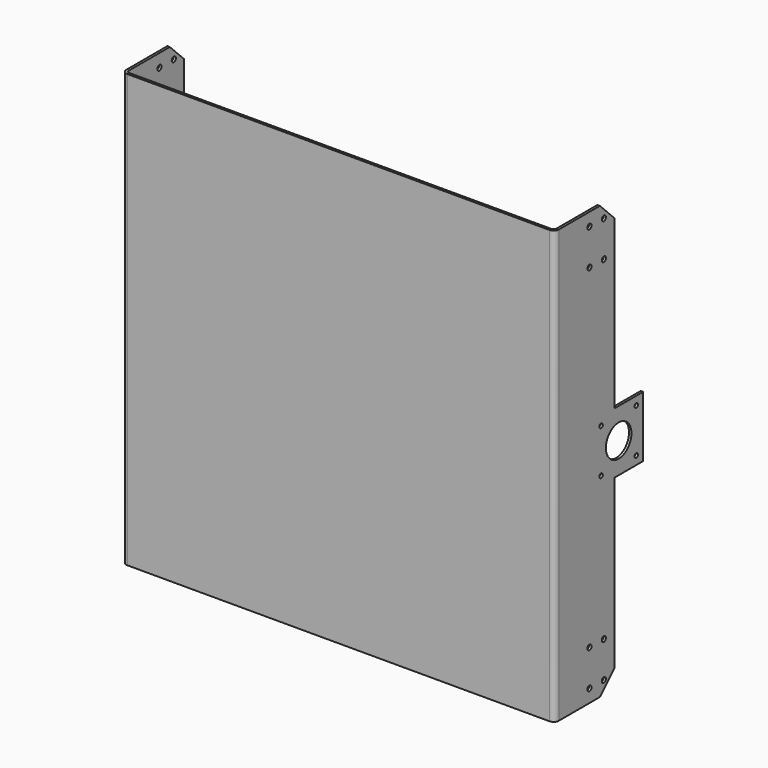
from build123d import *

# Parameters (mm, degrees)
F1_DEPTH  = 304.8
F2_R      = 3.69316
F3_R      = 1.98374
F4_W      = 1.70942
F4_H      = 43.0059846
F5_DEPTH  = 25.4
F6_R      = 11.2530001
F6_R_2    = 1.5
F7_DEPTH  = 1.70942
F8_SIZE   = 12.7
F9_R      = 1.8288
F10_DEPTH = 304.8


with BuildPart() as f1:
    # F0 (on Top) → F1 (new body)
    with BuildSketch(Plane.XY):
        Polygon((0, 50.8), (0, 0), (-301.38116, 0), (-301.38116, 50.8), (-303.09058, 50.8), (-303.09058, -1.70942), (1.70942, -1.70942), (1.70942, 50.8), align=None)
    extrude(amount=F1_DEPTH)

    # F2
    f2_edges = [f1.edges().sort_by_distance(p)[0] for p in [
        (1.70942, -1.70942, 152.4),
        (-303.09058, -1.70942, 152.4),
    ]]
    fillet(f2_edges, radius=F2_R)

    # F3
    f3_edges = [f1.edges().sort_by_distance(p)[0] for p in [
        (0, 0, 152.4),
        (-301.38116, 0, 152.4),
    ]]
    fillet(f3_edges, radius=F3_R)

    # F4 (on face) → F5 (join)
    with BuildSketch(Plane(origin=(0, 50.8, 0), x_dir=(-1, 0, 0), z_dir=(0, 1, 0))):
        with Locations((-0.85471, 152.4)):
            Rectangle(F4_W, F4_H)
    extrude(amount=F5_DEPTH)

    # F6 (on face) → F7 (cut, through all)
    with BuildSketch(Plane.YZ.offset(1.70942)):
        with Locations((54.6970077, 152.4)):
            Circle(F6_R)
        with Locations((70.1970021, 136.9000056)):
            Circle(F6_R_2)
        with Locations((39.1970133, 136.9000056)):
            Circle(F6_R_2)
        with Locations((39.1970133, 167.8999944)):
            Circle(F6_R_2)
        with Locations((70.1970021, 167.8999944)):
            Circle(F6_R_2)
    extrude(amount=-F7_DEPTH, mode=Mode.SUBTRACT)

    # F8
    f8_edges = [f1.edges().sort_by_distance(p)[0] for p in [
        (0.85471, 50.8, 0),
        (-302.23587, 50.8, 0),
        (-302.23587, 50.8, 304.8),
        (0.85471, 50.8, 304.8),
    ]]
    chamfer(f8_edges, length=F8_SIZE)

    # F9 (on face) → F10 (cut, through all)
    with BuildSketch(Plane.YZ.offset(1.70942)):
        with Locations((41.6436699622, 295.6436699622)):
            Circle(F9_R)
        with Locations((41.6436699622, 270.2436699622)):
            Circle(F9_R)
        with Locations((28.9436699622, 270.2436699622)):
            Circle(F9_R)
        with Locations((28.9436699622, 295.6436699622)):
            Circle(F9_R)
        with Locations((41.6436699622, 34.5563300378)):
            Circle(F9_R)
        with Locations((41.6436699622, 9.1563300378)):
            Circle(F9_R)
        with Locations((28.9436699622, 9.1563300378)):
            Circle(F9_R)
        with Locations((28.9436699622, 34.5563300378)):
            Circle(F9_R)
    extrude(amount=-F10_DEPTH, mode=Mode.SUBTRACT)


solid = f1.part
